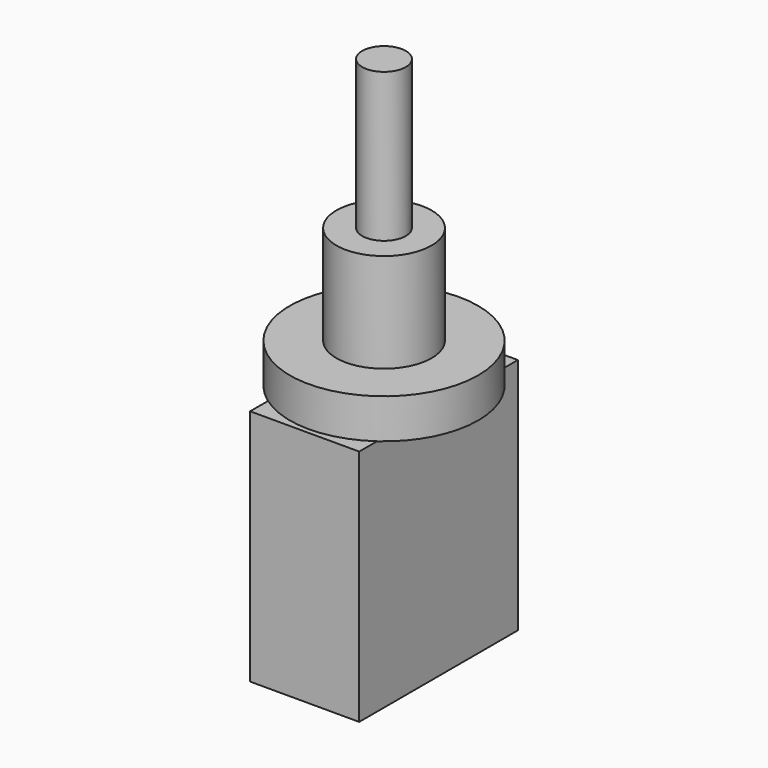
from build123d import *

# Parameters (mm, degrees)
F0_R     = 3.048
F1_DEPTH = 6.35
F2_R     = 6.0325
F2_R_2   = 3.048
F3_DEPTH = 2.54
F5_DEPTH = 15.24
F6_R     = 1.397
F7_DEPTH = 9.525


with BuildPart() as f1:
    # F0 (on Top) → F1 (new body)
    with BuildSketch(Plane.XY):
        Circle(F0_R)
    extrude(amount=F1_DEPTH)

    # F2 (on face) → F3 (join)
    with BuildSketch(Plane(origin=(0, 0, 0), x_dir=(1, 0, 0), z_dir=(0, 0, -1))):
        Circle(F2_R)
        Circle(F2_R_2, mode=Mode.SUBTRACT)
        Circle(F2_R_2)
    extrude(amount=F3_DEPTH)

    # F4 (on face) → F5 (join)
    with BuildSketch(Plane(origin=(0, 0, -2.54), x_dir=(1, 0, 0), z_dir=(0, 0, -1))):
        Polygon((3.4925, -6.35), (-3.4925, 6.35), (-3.4925, -6.35), align=None)
        Polygon((3.4925, 6.35), (-3.4925, 6.35), (3.4925, -6.35), align=None)
    extrude(amount=F5_DEPTH)

    # F6 (on face) → F7 (join)
    with BuildSketch(Plane.XY.offset(6.35)):
        Circle(F6_R)
    extrude(amount=F7_DEPTH)


solid = f1.part
